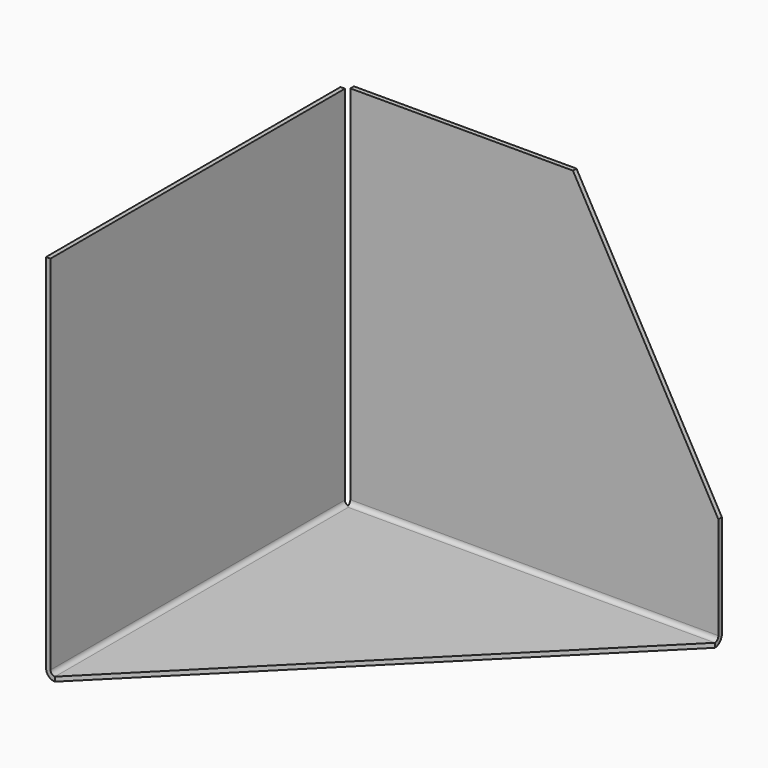
from build123d import *

# Parameters (mm, degrees)
F0_W        = 101.2
F0_H        = 101.2
F1_DEPTH    = 100
F2_T        = -1.2
F4_W        = 0.8
F4_H        = 0.8
F5_DEPTH    = 100.001
F6_R        = 1.2
F7_T4_DEPTH = 101.8
F8_R        = 2.4
F9_T1_DEPTH = 110.8
F12_DEPTH   = 25
F14_DEPTH   = 25


# Not quite as in the source:
# - a fillet or chamfer that OpenCascade refuses, or shapes differently, is made with other operations: its cross-section is extruded or revolved along the edge and cut away or added


with BuildPart() as f1:
    # F0 (on Top) → F1 (new body)
    with BuildSketch(Plane.XY):
        Rectangle(F0_W, F0_H)
    extrude(amount=F1_DEPTH)

    # F2
    f2_openings = [f1.faces().sort_by_distance(p)[0] for p in [
        (0, 0, 100),
        (0, -50.6, 50),
        (50.6, 0, 50),
    ]]
    offset(amount=F2_T, openings=f2_openings)

    # F4 (on face) → F5 (cut, through all)
    with BuildSketch(Plane.XY.offset(100)):
        with Locations((-49, 49)):
            Rectangle(F4_W, F4_H)
        Polygon((-50.6, 50.6), (-50.6, 48.6), (-49.4, 48.6), (-49.4, 49.4), (-48.6, 49.4), (-48.6, 50.6), align=None)
    extrude(amount=-F5_DEPTH, mode=Mode.SUBTRACT)

    # F6
    f6_edges = [f1.edges().sort_by_distance(p)[0] for p in [
        (1, 49.4, 1.2),
    ]]
    fillet(f6_edges, radius=F6_R)

    # F7: fillet of radius 1.2 on 1 edges, made by hand


with BuildPart() as f7_tool2:
    # F7_s3 → F7_t4 (new body)
    with BuildSketch(Plane.XZ.offset(50.6)):
        with BuildLine():
            ThreePointArc((-49.4, 2.4), (-49.0485281374, 1.5514718626), (-48.2, 1.2))
            Line((-48.2, 1.2), (-49.4, 1.2))
            Line((-49.4, 1.2), (-49.4, 2.4))
        make_face()
    extrude(amount=-F7_T4_DEPTH)

    split(bisect_by=Plane.XZ.offset(-48.6), keep=Keep.TOP)


with BuildPart() as f1_1:
    add(f1.part)

    # F7_t1: union F7_tool2
    add(f7_tool2.part)

    # F8
    f8_edges = [f1_1.edges().sort_by_distance(p)[0] for p in [
        (-50.6, -1, 0),
    ]]
    fillet(f8_edges, radius=F8_R)

    # F9: fillet of radius 2.4 on 1 edges, made by hand

    # F9_s2 → F9_t1 (cut)
    with BuildSketch(Plane.YZ.offset(-54.2)):
        with BuildLine():
            ThreePointArc((50.6, 2.4), (49.8970562748, 0.7029437252), (48.2, 0))
            Line((48.2, 0), (50.6, 0))
            Line((50.6, 0), (50.6, 2.4))
        make_face()
    extrude(amount=F9_T1_DEPTH, mode=Mode.SUBTRACT)

    # F11 (on face) → F12 (cut)
    with BuildSketch(Plane(origin=(0, 50.6, 0), x_dir=(-1, 0, 0), z_dir=(0, 1, 0))):
        Polygon((-11.4, 100), (-50.6, 100), (-50.6, 30), align=None)
    extrude(amount=-F12_DEPTH, mode=Mode.SUBTRACT)

    # F13 (on face) → F14 (cut)
    with BuildSketch(Plane(origin=(0, 0, 0), x_dir=(1, 0, 0), z_dir=(0, 0, -1))):
        Polygon((50.6, -48.2), (50.6, 50.6), (-48.2, 50.6), align=None)
    extrude(amount=-F14_DEPTH, mode=Mode.SUBTRACT)


solid = f1_1.part
